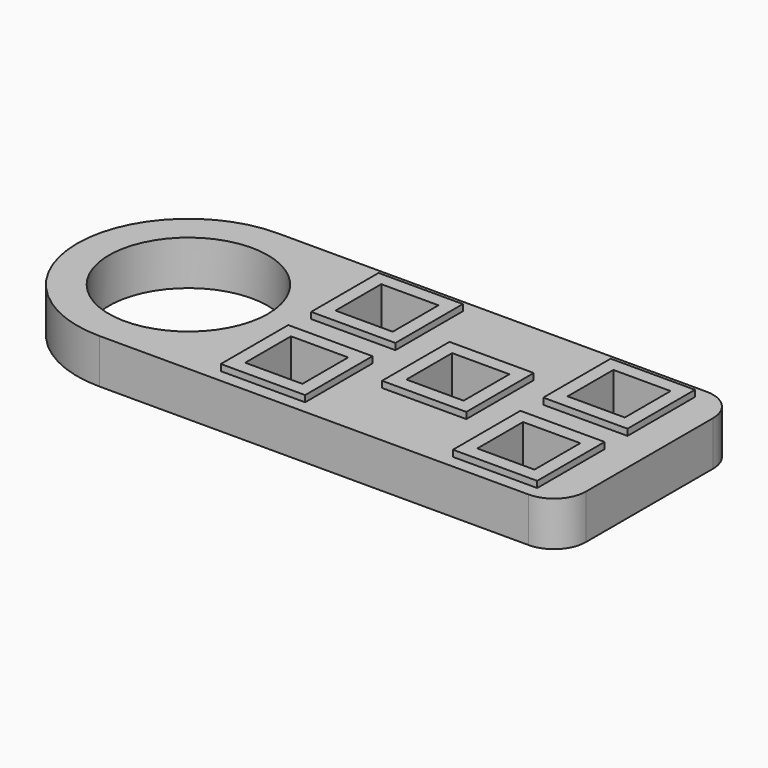
from build123d import *

# Parameters (mm, degrees)
F0_R         = 12.5
F1_DEPTH     = 7
F2_W         = 13.25
F2_H         = 13.25
F2_W_2       = 9
F2_H_2       = 9
F3_DEPTH     = 1
F4_DEPTH     = 5
F5_TEXT_SIZE = 5.5555555556
F6_DEPTH     = 1


# Not quite as in the source:
# - Text() gives the source's letters only with a copy of the font that has no kerning and outlines rounded to 1/6400 em; it was checked with that copy


with BuildPart() as f1:
    # F0 (on Top) → F1 (new body)
    with BuildSketch(Plane.XY):
        with BuildLine():
            ThreePointArc((0, 17.5), (5.1256313292, 5.1256313292), (17.5, 0))
            Line((17.5, 0), (85, 0))
            ThreePointArc((85, 0), (88.5355339059, 1.4644660941), (90, 5))
            Line((90, 5), (90, 30))
            ThreePointArc((90, 30), (88.5355339059, 33.5355339059), (85, 35))
            Line((85, 35), (17.5, 35))
            ThreePointArc((17.5, 35), (5.1256313292, 29.8743686708), (0, 17.5))
        make_face()
        with Locations((17.5, 17.5)):
            Circle(F0_R, mode=Mode.SUBTRACT)
    extrude(amount=F1_DEPTH)

    # F2 (on face) → F3 (join)
    with BuildSketch(Plane.XY.offset(7)):
        with Locations((41.625, 26.375)):
            Rectangle(F2_W, F2_H)
        with Locations((41.625, 26.375)):
            Rectangle(F2_W_2, F2_H_2, mode=Mode.SUBTRACT)
        with Locations((41.625, 8.625)):
            Rectangle(F2_W, F2_H)
        with Locations((41.625, 8.625)):
            Rectangle(F2_W_2, F2_H_2, mode=Mode.SUBTRACT)
        with Locations((59.875, 17.5)):
            Rectangle(F2_W, F2_H)
        with Locations((59.875, 17.5)):
            Rectangle(F2_W_2, F2_H_2, mode=Mode.SUBTRACT)
        with Locations((78.125, 8.625)):
            Rectangle(F2_W, F2_H)
        with Locations((78.125, 8.625)):
            Rectangle(F2_W_2, F2_H_2, mode=Mode.SUBTRACT)
        with Locations((78.125, 26.375)):
            Rectangle(F2_W, F2_H)
        with Locations((78.125, 26.375)):
            Rectangle(F2_W_2, F2_H_2, mode=Mode.SUBTRACT)
    extrude(amount=F3_DEPTH)

    # F2 (on face) → F4 (cut)
    with BuildSketch(Plane.XY.offset(7)):
        with Locations((41.625, 26.375)):
            Rectangle(F2_W_2, F2_H_2)
        with Locations((41.625, 8.625)):
            Rectangle(F2_W_2, F2_H_2)
        with Locations((59.875, 17.5)):
            Rectangle(F2_W_2, F2_H_2)
        with Locations((78.125, 26.375)):
            Rectangle(F2_W_2, F2_H_2)
        with Locations((78.125, 8.625)):
            Rectangle(F2_W_2, F2_H_2)
    extrude(amount=-F4_DEPTH, mode=Mode.SUBTRACT)

    # F5 (on face) → F6 (cut)
    with BuildSketch(Plane(origin=(0, 0, 0), x_dir=(1, 0, 0), z_dir=(0, 0, -1))):
        with Locations((30, -9)):
            Text('910, 911', F5_TEXT_SIZE, font='Open Sans', text_align=(TextAlign.LEFT, TextAlign.BOTTOM))
    extrude(amount=-F6_DEPTH, mode=Mode.SUBTRACT)


solid = f1.part
